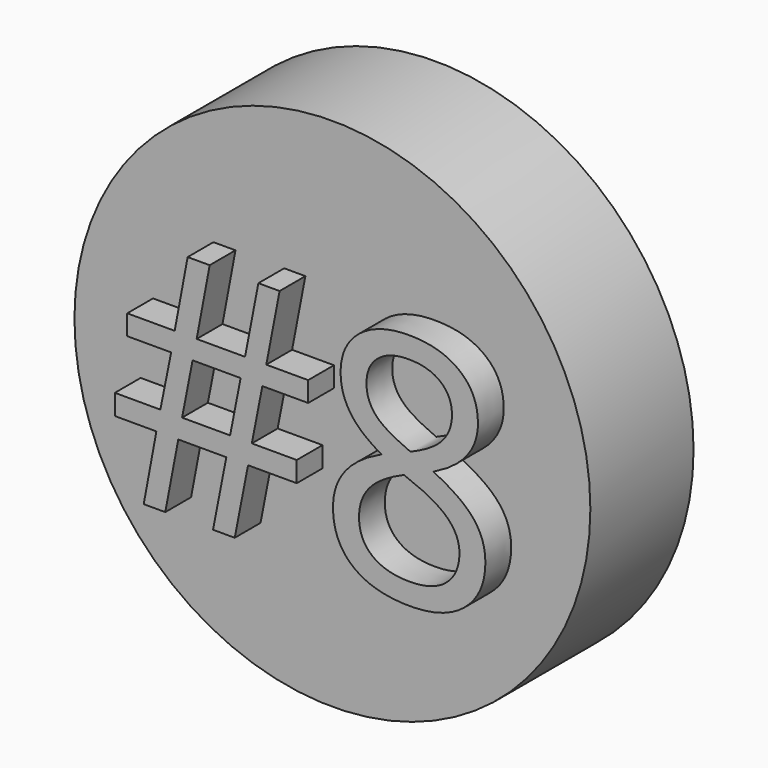
from build123d import *

# Parameters (mm, degrees)
F0_R         = 50.8
F1_DEPTH     = 25.4
F2_TEXT_SIZE = 63.9444010125
F3_DEPTH     = 6.35


# Not quite as in the source:
# - Text() gives the source's letters only with a copy of the font that has no kerning and outlines rounded to 1/6400 em; it was checked with that copy


with BuildPart() as f1:
    # F0 (on Front) → F1 (new body)
    with BuildSketch(Plane.XZ):
        Circle(F0_R)
    extrude(amount=F1_DEPTH)

    # F2 (on face) → F3 (join)
    with BuildSketch(Plane.XZ.offset(25.4)):
        with Locations((-39.3507849043, -23.5177148134)):
            Text('#8', F2_TEXT_SIZE, font='Open Sans', text_align=(TextAlign.LEFT, TextAlign.BOTTOM))
    extrude(amount=F3_DEPTH)


solid = f1.part
